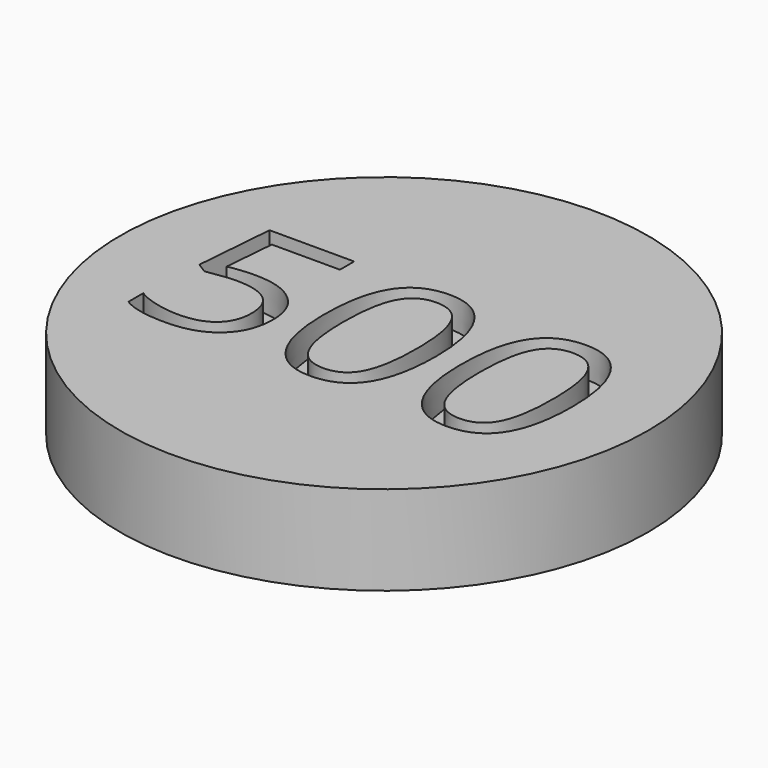
from build123d import *

# Parameters (mm, degrees)
F0_R         = 9.75
F1_DEPTH     = 3.302
F2_TEXT_SIZE = 8.8076575763
F3_DEPTH     = 1.1176


# Not quite as in the source:
# - Text() gives the source's letters only with a copy of the font that has no kerning and outlines rounded to 1/6400 em; it was checked with that copy


with BuildPart() as f1:
    # F0 (on Top) → F1 (new body)
    with BuildSketch(Plane.XY):
        Circle(F0_R)
    extrude(amount=F1_DEPTH)

    # F2 (on face) → F3 (cut)
    with BuildSketch(Plane.XY.offset(3.302)):
        with Locations((-7.5577439748, -3.3288064021)):
            Text('500', F2_TEXT_SIZE, font='Open Sans', text_align=(TextAlign.LEFT, TextAlign.BOTTOM))
    extrude(amount=-F3_DEPTH, mode=Mode.SUBTRACT)


solid = f1.part
